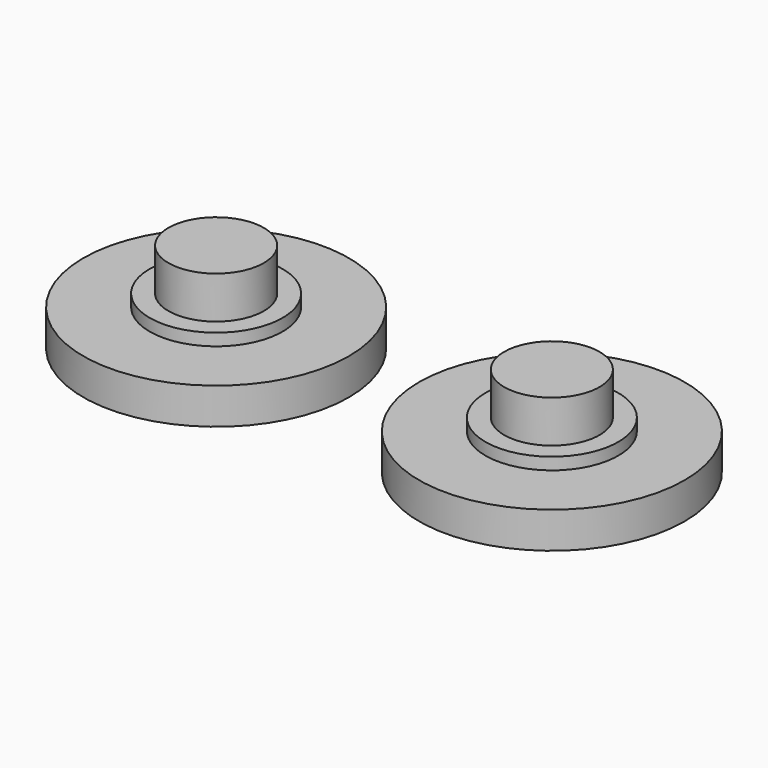
from build123d import *

# Parameters (mm, degrees)
F4_TEXT_SIZE = 18.0042064231
F6_DEPTH     = 0.25
F5_TEXT_SIZE = 20.8222559498
F7_DEPTH     = 0.25


# Not quite as in the source:
# - Text() gives the source's letters only with a copy of the font that has no kerning and outlines rounded to 1/6400 em; it was checked with that copy


with BuildPart() as f2:
    # F0 (on Front) → F2 (revolve)
    with BuildSketch(Plane.XZ):
        Polygon((0, 0), (0, 7.5), (-3.95, 7.5), (-3.95, 4), (-5.5, 4), (-5.5, 3), (-11, 3), (-11, 0), align=None)
    revolve(axis=Axis((0, 0, 3.75), (0, 0, 1)))

    # F5 (on face) → F7 (cut)
    with BuildSketch(Plane(origin=(0, 0, 0), x_dir=(1, 0, 0), z_dir=(0, 0, -1))):
        with Locations((-6.1654476449, -7.0193153806)):
            Text('E', F5_TEXT_SIZE, font='Open Sans', text_align=(TextAlign.LEFT, TextAlign.BOTTOM))
    extrude(amount=-F7_DEPTH, mode=Mode.SUBTRACT)


with BuildPart() as f3:
    # F1 (on Front) → F3 (revolve)
    with BuildSketch(Plane.XZ):
        Polygon((-38.8061414476, 0), (-27.8061414476, 0), (-27.8061414476, 7.5), (-31.7561414476, 7.5), (-31.7561414476, 4), (-33.3061414476, 4), (-33.3061414476, 3), (-38.8061414476, 3), align=None)
    revolve(axis=Axis((-27.8061414476, 0, 3.75), (0, 0, 1)))

    # F4 (on face) → F6 (cut)
    with BuildSketch(Plane(origin=(0, 0, 0), x_dir=(1, 0, 0), z_dir=(0, 0, -1))):
        with Locations((-34.4586670399, -5.8920956217)):
            Text('R', F4_TEXT_SIZE, font='Open Sans', text_align=(TextAlign.LEFT, TextAlign.BOTTOM))
    extrude(amount=-F6_DEPTH, mode=Mode.SUBTRACT)


solid = Compound([f2.part, f3.part])
